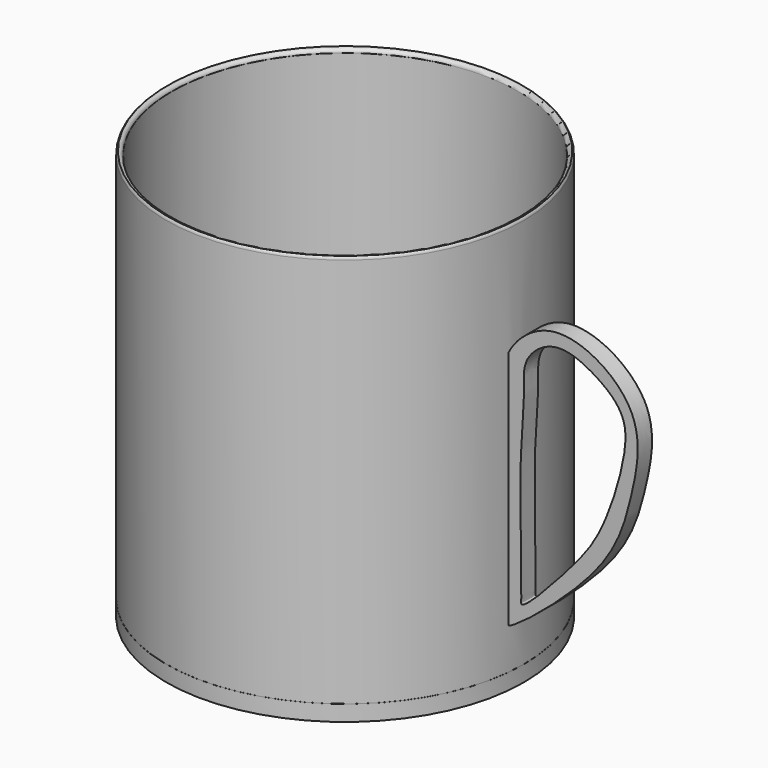
from build123d import *

# Parameters (mm, degrees)
F0_R     = 45
F1_DEPTH = 4
F2_R     = 44.9761258013
F2_R_2   = 43.629041266
F3_DEPTH = 99
F4_R     = 1
F7_DEPTH = 4.5


# Not quite as in the source:
# - a fillet or chamfer that OpenCascade refuses, or shapes differently, is made with other operations: its cross-section is extruded or revolved along the edge and cut away or added


with BuildPart() as f1:
    # F0 (on Top) → F1 (new body)
    with BuildSketch(Plane.XY):
        Circle(F0_R)
    extrude(amount=F1_DEPTH)

    # F2 (on face) → F3 (join)
    with BuildSketch(Plane.XY.offset(4)):
        Circle(F2_R)
        Circle(F2_R_2, mode=Mode.SUBTRACT)
    extrude(amount=F3_DEPTH)

    # F4
    f4_edges = [f1.edges().sort_by_distance(p)[0] for p in [
        (-43.629041, 0, 103),
    ]]
    fillet(f4_edges, radius=F4_R)

    # F5: fillet of radius 1 on 1 edges, made by hand

    # F5_s1 → F5_t2 (revolve, cut)
    with BuildSketch(Plane.XZ):
        with BuildLine():
            ThreePointArc((44.629041266, 103), (44.8852230086, 102.6591532601), (44.9761258013, 102.2425692137))
            Line((44.9761258013, 102.2425692137), (44.9761258013, 103))
            Line((44.9761258013, 103), (44.629041266, 103))
        make_face()
    revolve(axis=Axis((0, 0, 103), (0, 0, 1)), mode=Mode.SUBTRACT)

    # F6 (on Front) → F7 (join)
    with BuildSketch(Plane.XZ):
        with BuildLine():
            add(Edge.make_bspline(
                [(44.6038767695, 74.4961425662), (46.058109389, 77.8182076206), (55.8368160451, 88.024936908), (79.9742466822, 73.8892972273), (75.5578302702, 51.8870499933), (70.2818798321, 33.5907882729), (44.0965457743, 12.4948044006), (44.472748151, 15.4069988545), (44.1140623698, 20.3831180198), (44.5373091257, 31.8060604461), (43.8121190937, 59.7639995048), (44.1850678129, 68.8259472254), (43.7065695005, 72.4463239322), (44.6038767695, 74.4961425662)],
                knots=[0, 0, 0, 0, 0.0942351755, 0.2113427888, 0.3208435248, 0.4391747045, 0.5719407491, 0.5939885781, 0.6467857692, 0.733817392, 0.8669260561, 0.9418539325, 1, 1, 1, 1], degree=3))
        make_face()
        with BuildLine():
            add(Edge.make_bspline(
                [(48.0379648507, 20.0913008302), (49.0473035571, 19.7528414427), (61.179570465, 32.7730244456), (68.6340461757, 42.4827654099), (74.5036345483, 61.3892931083), (74.1615493778, 70.8476949562), (66.7393547532, 77.1429330303), (56.3676694437, 81.7412992572), (48.008237042, 74.9677614325), (48.9209394578, 67.10815582), (47.6541737083, 55.1398660778), (47.7173765122, 42.0433803787), (47.817758942, 32.6512806631), (47.8283403305, 22.9375669913), (47.9753912955, 21.4638792573), (47.7683357752, 20.1817149709), (48.0379648507, 20.0913008302)],
                knots=[0, 0, 0, 0, 0.0931226593, 0.1850581318, 0.286254836, 0.3554844297, 0.4259177612, 0.5019638348, 0.5706279296, 0.6339488651, 0.7154899004, 0.8001557754, 0.8748024428, 0.9452073859, 0.9751237356, 1, 1, 1, 1], degree=3))
        make_face(mode=Mode.SUBTRACT)
    extrude(amount=F7_DEPTH)


solid = f1.part
